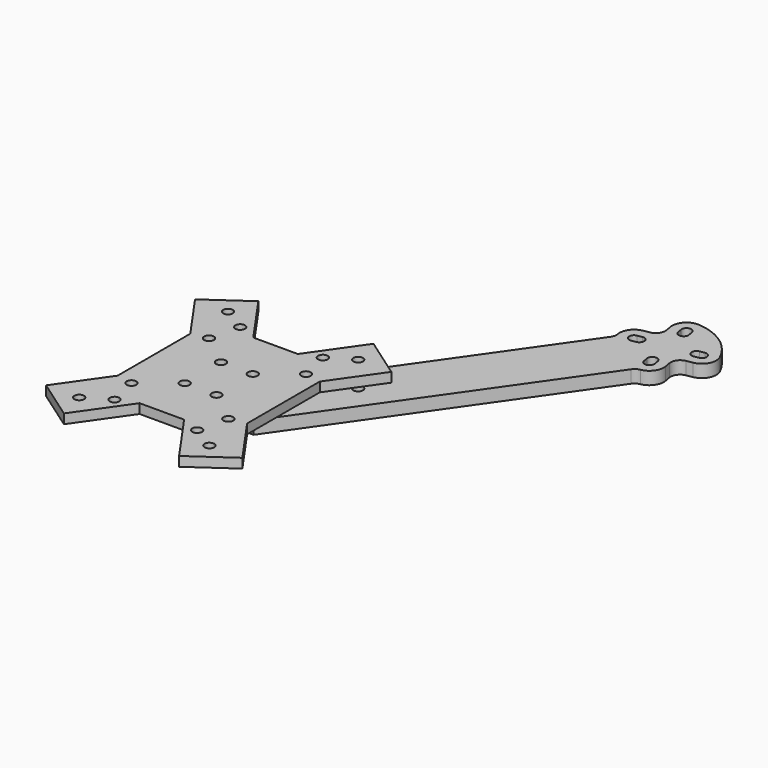
from build123d import *

# Parameters (mm, degrees)
F0_R     = 1.525
F1_DEPTH = 4
F3_R     = 1.525
F4_DEPTH = 3


# Not quite as in the source:
# - a feature names something its author has since deleted; it is built from what else it names


with BuildPart() as f1:
    # F0 (on Top) → F1 (new body)
    with BuildSketch(Plane.XY):
        with BuildLine():
            Line((51.6620058257, 89.4720118049), (0, 15.6910211606))
            Line((0, 15.6910211606), (0, 0))
            Line((0, 0), (10.9869712989, 0))
            Line((10.9869712989, 0), (66.4067426229, 79.1476359506))
            ThreePointArc((66.4067426229, 79.1476359506), (67.261429469, 79.9628740335), (68.3645638504, 80.3850082222))
            ThreePointArc((68.3645638504, 80.3850082222), (71.3082325233, 82.2380356387), (72.0672029506, 85.6325694436))
            Line((72.0672029506, 85.6325694436), (71.7242477997, 87.5775647558))
            ThreePointArc((71.7242477997, 87.5775647558), (72.2212149259, 89.8192385978), (74.1577265257, 91.0529325478))
            Line((74.1577265257, 91.0529325478), (76.1027218379, 91.3958876987))
            ThreePointArc((76.1027218379, 91.3958876987), (79.3253389122, 93.7524870397), (79.4277203932, 97.743519399))
            ThreePointArc((79.4277203932, 97.743519399), (73.452695276, 104.9013203483), (64.682983596, 108.0678952533))
            ThreePointArc((64.682983596, 108.0678952533), (60.9676564674, 106.6066746716), (59.8553774102, 102.7724007429))
            Line((59.8553774102, 102.7724007429), (60.198332561, 100.8274054307))
            ThreePointArc((60.198332561, 100.8274054307), (59.7013654349, 98.5857315887), (57.764853835, 97.3520376387))
            Line((57.764853835, 97.3520376387), (55.8198585228, 97.0090824878))
            ThreePointArc((55.8198585228, 97.0090824878), (52.8896233297, 95.1348846394), (52.1551411217, 91.7349682069))
            ThreePointArc((52.1551411217, 91.7349682069), (52.1357589189, 90.5539825732), (51.6620058257, 89.4720118049))
        make_face()
        with Locations((5, 7.1407400337)):
            Circle(F0_R, mode=Mode.SUBTRACT)
        with Locations((12.9988775531, 24.7099710219)):
            Circle(F0_R, mode=Mode.SUBTRACT)
        with Locations((20.475, 29.241330438)):
            Circle(F0_R, mode=Mode.SUBTRACT)
        with BuildLine():
            Line((56.3408030558, 94.0546592287), (57.8180146853, 94.3151314952))
            ThreePointArc((57.8180146853, 94.3151314952), (59.5846599796, 93.0781131428), (58.3476416272, 91.3114678486))
            Line((58.3476416272, 91.3114678486), (56.8704299977, 91.0509955821))
            ThreePointArc((56.8704299977, 91.0509955821), (55.1037847034, 92.2880139345), (56.3408030558, 94.0546592287))
        make_face(mode=Mode.SUBTRACT)
        with BuildLine():
            Line((66.1091160449, 84.5819979687), (65.8486437784, 86.0592095982))
            ThreePointArc((65.8486437784, 86.0592095982), (67.0856621308, 87.8258548925), (68.852307425, 86.5888365401))
            Line((68.852307425, 86.5888365401), (69.1127796915, 85.1116249106))
            ThreePointArc((69.1127796915, 85.1116249106), (67.8757613391, 83.3449796163), (66.1091160449, 84.5819979687))
        make_face(mode=Mode.SUBTRACT)
        with BuildLine():
            ThreePointArc((66.0739365824, 102.3457605883), (64.83691823, 100.579115294), (63.0702729357, 101.8161336464))
            Line((63.0702729357, 101.8161336464), (62.8098006692, 103.2933452759))
            ThreePointArc((62.8098006692, 103.2933452759), (64.0468190216, 105.0599905702), (65.8134643159, 103.8229722178))
            Line((65.8134643159, 103.8229722178), (66.0739365824, 102.3457605883))
        make_face(mode=Mode.SUBTRACT)
        with BuildLine():
            ThreePointArc((74.1045656754, 94.0898386912), (72.3379203811, 95.3268570436), (73.5749387335, 97.0935023379))
            Line((73.5749387335, 97.0935023379), (75.052150363, 97.3539746044))
            ThreePointArc((75.052150363, 97.3539746044), (76.8187956573, 96.116956252), (75.5817773049, 94.3503109577))
            Line((75.5817773049, 94.3503109577), (74.1045656754, 94.0898386912))
        make_face(mode=Mode.SUBTRACT)
    extrude(amount=F1_DEPTH)


with BuildPart() as f4:
    # F3 (on offset) → F4 (new body)
    with BuildSketch(Plane.XY.offset(9)):
        Polygon((30.8714845867, 29.2862810921), (18.1126643716, 38.2201031854), (7.0020753821, 22.3525376663), (0, 22.3525376663), (-7.0020753821, 22.3525376663), (-18.1126643716, 38.2201031854), (-30.8714845867, 29.2862810921), (-20.3650097999, 14.2814800674), (-20.3650097999, 0), (-20.3650097999, -14.2814800674), (-30.8714845867, -29.2862810921), (-18.1126643716, -38.2201031854), (-7.0020753821, -22.3525376663), (0, -22.3525376663), (7.0020753821, -22.3525376663), (18.1126643716, -38.2201031854), (30.8714845867, -29.2862810921), (20.3650097999, -14.2814800674), (20.3650097999, 0), (20.3650097999, 14.2814800674), align=None)
        with Locations((-20.475, -29.241330438)):
            Circle(F3_R, mode=Mode.SUBTRACT)
        with Locations((-12.9988775531, -24.7099710219)):
            Circle(F3_R, mode=Mode.SUBTRACT)
        with Locations((-15.25, -15.25)):
            Circle(F3_R, mode=Mode.SUBTRACT)
        with Locations((-5, -7.1407400337)):
            Circle(F3_R, mode=Mode.SUBTRACT)
        with Locations((12.9988775531, -24.7099710219)):
            Circle(F3_R, mode=Mode.SUBTRACT)
        with Locations((20.475, -29.241330438)):
            Circle(F3_R, mode=Mode.SUBTRACT)
        with Locations((15.25, -15.25)):
            Circle(F3_R, mode=Mode.SUBTRACT)
        with Locations((5, -7.1407400337)):
            Circle(F3_R, mode=Mode.SUBTRACT)
        with Locations((-5, 7.1407400337)):
            Circle(F3_R, mode=Mode.SUBTRACT)
        with Locations((-15.25, 15.25)):
            Circle(F3_R, mode=Mode.SUBTRACT)
        with Locations((-20.475, 29.241330438)):
            Circle(F3_R, mode=Mode.SUBTRACT)
        with Locations((-12.9988775531, 24.7099710219)):
            Circle(F3_R, mode=Mode.SUBTRACT)
        with Locations((5, 7.1407400337)):
            Circle(F3_R, mode=Mode.SUBTRACT)
        with Locations((15.25, 15.25)):
            Circle(F3_R, mode=Mode.SUBTRACT)
        with Locations((12.9988775531, 24.7099710219)):
            Circle(F3_R, mode=Mode.SUBTRACT)
        with Locations((20.475, 29.241330438)):
            Circle(F3_R, mode=Mode.SUBTRACT)
    extrude(amount=F4_DEPTH)


solid = Compound([f1.part, f4.part])
